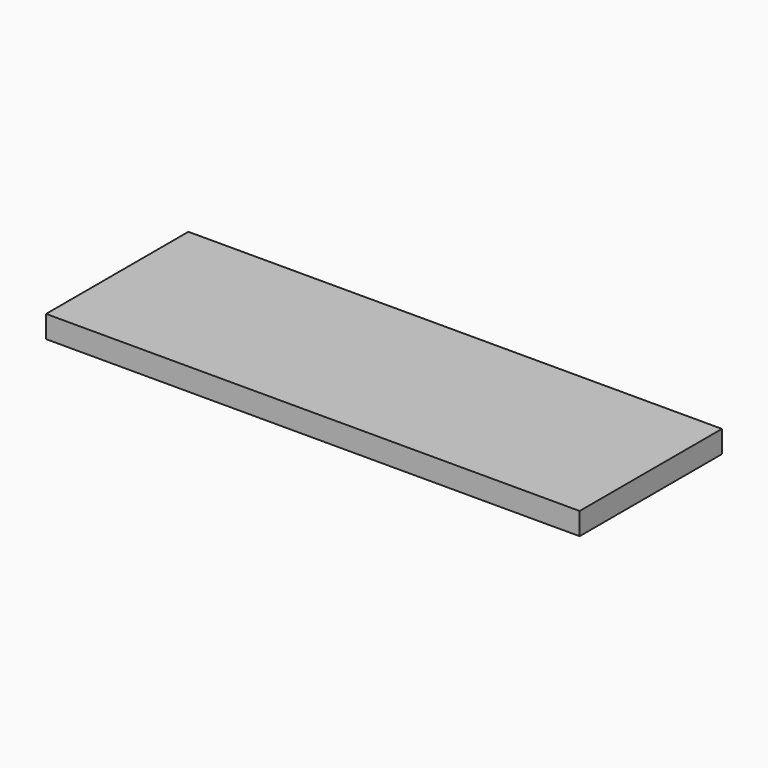
from build123d import *

# Parameters (mm, degrees)
F0_W     = 76.2
F0_H     = 25.4
F1_DEPTH = 3.175


# Not quite as in the source:
# - a length typed as a fraction of an inch, garbled in the dataset ("3 / 203.2 mm" for 3/8 in), is restored


with BuildPart() as f1:
    # F0 (on Top) → F1 (new body)
    with BuildSketch(Plane.XY):
        Rectangle(F0_W, F0_H)
    extrude(amount=F1_DEPTH)


solid = f1.part
